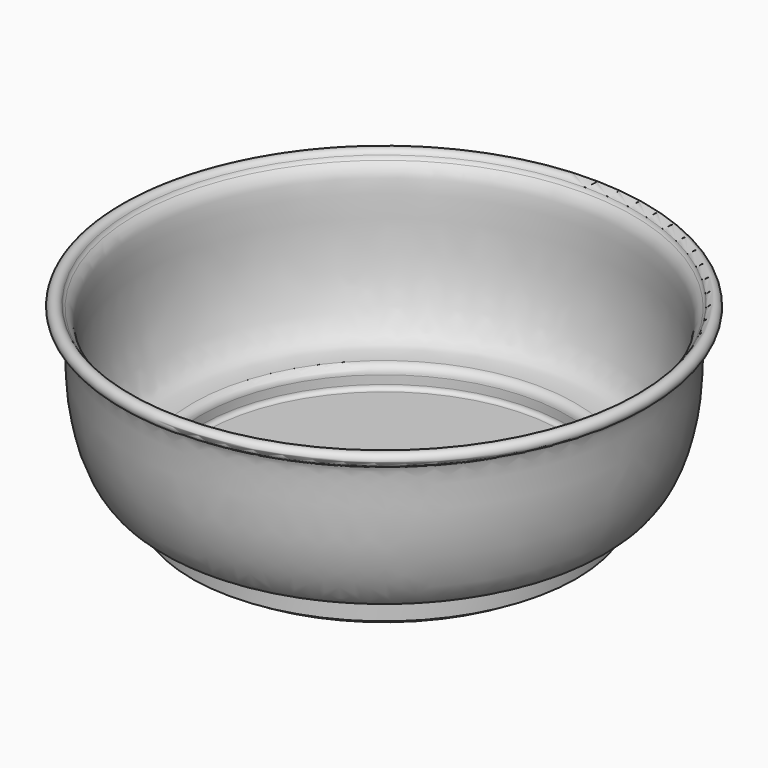
from build123d import *

# Parameters (mm, degrees)
F2_R     = 1
F3_R     = 42.5
F4_DEPTH = 1.5


# Not quite as in the source:
# - ends of sketch curves that miss each other by under 0.0002 mm in the source are joined
# - the dataset's text gives a spline's control points without its knots; the knots are read off the source's solid


with BuildPart() as f1:
    # F0 (on Front) → F1 (revolve)
    with BuildSketch(Plane.XZ):
        with BuildLine():
            Line((0, 2), (0, 0))
            Line((0, 0), (45, 0))
            Line((45, 0), (45, 4.1077052209))
            ThreePointArc((45, 4.1077052209), (45.251607634, 4.770961481), (45.8798177332, 5.1004570644))
            add(Edge.make_bspline(
                [(59.117932503, 39.1061978883), (58.9984398686, 38.9167118255), (57.961379378, 36.7467385449), (59.1133721589, 22.9753032204), (53.6275212518, 6.4619991243), (47.9608297571, 5.3523838112), (45.8798177332, 5.1004570644)],
                knots=[0.079529872, 0.079529872, 0.079529872, 0.079529872, 0.1164806675, 0.435781553, 0.7789347917, 0.9727324769, 0.9727324769, 0.9727324769, 0.9727324769], degree=3))
            ThreePointArc((59.117932503, 39.1061978883), (59.7042053248, 39.7061118302), (60.4849287438, 40.0128421715))
            ThreePointArc((60.4849287438, 40.0128421715), (61.4445872468, 42.4401309197), (58.8691826, 42.0159069052))
            ThreePointArc((58.8691826, 42.0159069052), (58.643182834, 41.577442369), (58.31674753, 41.2076237072))
            add(Edge.make_bspline(
                [(58.31674753, 41.2076237072), (58.3148397341, 41.2059420359), (58.1329946532, 41.0449587485), (57.8276969018, 40.7452853769), (57.4453837385, 40.220259631), (57.1893214461, 39.771564073), (56.9743902421, 39.277445408), (56.8043597407, 38.7424234539), (56.680003708, 38.203859582), (56.5520410764, 37.4591588813), (56.4452689195, 36.4663757584), (56.3674656809, 35.155302403), (56.3050858948, 33.2523114152), (56.2634042278, 30.6110777497), (56.1735934989, 27.7415742893), (56.018450433, 25.3953023971), (55.8477339812, 23.6368985798), (55.6092469781, 21.8895853556), (55.2036356572, 19.5864432025), (54.539773, 16.8097339131), (53.5203746444, 13.7898979021), (52.5184171783, 11.6646836577), (51.6611889381, 10.2810715096), (51.1154343385, 9.5653431356), (50.6822443153, 9.0894464967), (50.3647724491, 8.7843429997), (50.0474792797, 8.5214792406), (49.6165481094, 8.2146567762), (49.059056291, 7.9027315772), (48.0980536701, 7.5169322584), (46.7280561328, 7.2056808972), (45.4526028209, 7.0623561488), (44.7798504425, 6.9878504754)],
                knots=[0.0309186802, 0.0309186802, 0.0309186802, 0.0309186802, 0.03125, 0.0625, 0.078125, 0.09375, 0.109375, 0.125, 0.140625, 0.15625, 0.1875, 0.21875, 0.25, 0.3125, 0.375, 0.40625, 0.4375, 0.46875, 0.5, 0.5625, 0.625, 0.6875, 0.71875, 0.75, 0.765625, 0.78125, 0.796875, 0.8125, 0.84375, 0.875, 0.9375, 1, 1, 1, 1], degree=3))
            ThreePointArc((44.7798504425, 6.9878504754), (43.5099827366, 6.3341112085), (42.9999989595, 5))
            Line((42.9999989595, 5), (42.9999994798, 2))
            Line((42.9999994798, 2), (0, 2))
        make_face()
    revolve(axis=Axis((0, 0, 20.8975244313), (0, 0, 1)))

    # F2
    f2_edges = [f1.edges().sort_by_distance(p)[0] for p in [
        (-42.999999, 0, 2),
    ]]
    fillet(f2_edges, radius=F2_R)

    # F3 (on face) → F4 (join)
    with BuildSketch(Plane(origin=(0, 0, 0), x_dir=(1, 0, 0), z_dir=(0, 0, -1))):
        Circle(F3_R)
    extrude(amount=F4_DEPTH)


solid = f1.part
